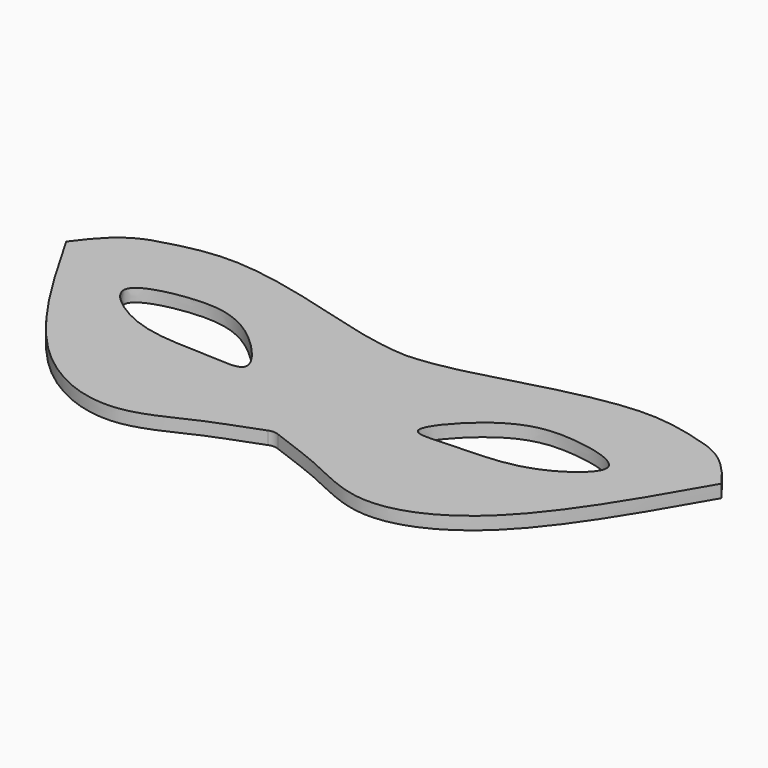
from build123d import *

# Parameters (mm, degrees)
F1_DEPTH = 2.54


with BuildPart() as f1:
    # F0 (on Top) → F1 (new body)
    with BuildSketch(Plane.XY):
        with BuildLine():
            add(Edge.make_bspline(
                [(-64.9001970887, 13.9585789293), (-59.8424235445, 21.0693185661), (-53.7346048637, 23.0257404726), (-40.3145630415, 26.4282743713), (-18.8814266067, 21.0659037421), (-6.7937120551, 17.3061378378), (0, 16.9809884228)],
                knots=[0, 0, 0, 0, 0.236178933, 0.4480704868, 0.7301373435, 1, 1, 1, 1], degree=3))
            add(Edge.make_bspline(
                [(-64.9001970887, 13.9585789293), (-60.7131418232, 6.874283925), (-47.3204689226, -18.4135182685), (-25.1756609398, -27.5932197086), (-12.0182650538, -19.6967941746), (-3.849485648, -17.1576407451), (-0.9746632453, -15.96304804)],
                knots=[0, 0, 0, 0, 0.3337918688, 0.5942910183, 0.8077332916, 0.9798868813, 0.9798868813, 0.9798868813, 0.9798868813], degree=3))
            add(Edge.make_bspline(
                [(-0.9746632453, -15.96304804), (-0.6387908173, -15.8234808959), (-0.3134590553, -15.6830816698), (0, -15.541062241)],
                knots=[0.9798868813, 0.9798868813, 0.9798868813, 0.9798868813, 1, 1, 1, 1], degree=3))
            add(Edge.make_bspline(
                [(0.9746632453, -15.96304804), (0.6387908173, -15.8234808959), (0.3134590553, -15.6830816698), (0, -15.541062241)],
                knots=[0.9798868813, 0.9798868813, 0.9798868813, 0.9798868813, 1, 1, 1, 1], degree=3))
            add(Edge.make_bspline(
                [(64.9001970887, 13.9585789293), (60.7131418232, 6.874283925), (47.3204689226, -18.4135182685), (25.1756609398, -27.5932197086), (12.0182650538, -19.6967941746), (3.849485648, -17.1576407451), (0.9746632453, -15.96304804)],
                knots=[0, 0, 0, 0, 0.3337918688, 0.5942910183, 0.8077332916, 0.9798868813, 0.9798868813, 0.9798868813, 0.9798868813], degree=3))
            add(Edge.make_bspline(
                [(64.9001970887, 13.9585789293), (59.8424235445, 21.0693185661), (53.7346048637, 23.0257404726), (40.3145630415, 26.4282743713), (18.8814266067, 21.0659037421), (6.7937120551, 17.3061378378), (0, 16.9809884228)],
                knots=[0, 0, 0, 0, 0.236178933, 0.4480704868, 0.7301373435, 1, 1, 1, 1], degree=3))
        make_face()
        with BuildLine():
            add(Edge.make_bspline(
                [(-47.7647706866, 7.2845630348), (-47.2238090705, 9.4418665585), (-36.443945915, 12.1785918421), (-25.3808361667, 10.3769526965), (-13.4196607123, -3.1638753962), (-24.0941982433, -1.8972065882), (-32.4275500412, -2.0995535899), (-41.7821849404, -0.0363742902), (-48.2414855386, 5.383469502), (-47.7647706866, 7.2845630348)],
                knots=[0, 0, 0, 0, 0.1486904868, 0.3142704588, 0.4735401823, 0.5857095329, 0.7237633974, 0.8689685898, 1, 1, 1, 1], degree=3))
        make_face(mode=Mode.SUBTRACT)
        with BuildLine():
            add(Edge.make_bspline(
                [(47.7647706866, 7.2845630348), (47.2238090705, 9.4418665585), (36.443945915, 12.1785918421), (25.3808361667, 10.3769526965), (13.4196607123, -3.1638753962), (24.0941982433, -1.8972065882), (32.4275500412, -2.0995535899), (41.7821849404, -0.0363742902), (48.2414855386, 5.383469502), (47.7647706866, 7.2845630348)],
                knots=[0, 0, 0, 0, 0.1486904868, 0.3142704588, 0.4735401823, 0.5857095329, 0.7237633974, 0.8689685898, 1, 1, 1, 1], degree=3))
        make_face(mode=Mode.SUBTRACT)
        with BuildLine():
            add(Edge.make_bspline(
                [(-0.9746632453, -15.96304804), (-0.6387908173, -15.8234808959), (-0.3134590553, -15.6830816698), (0, -15.541062241)],
                knots=[0.9798868813, 0.9798868813, 0.9798868813, 0.9798868813, 1, 1, 1, 1], degree=3))
            ThreePointArc((-0.9746632453, -15.96304804), (0, -15.7686037435), (0.9746632453, -15.96304804))
            add(Edge.make_bspline(
                [(0.9746632453, -15.96304804), (0.6387908173, -15.8234808959), (0.3134590553, -15.6830816698), (0, -15.541062241)],
                knots=[0.9798868813, 0.9798868813, 0.9798868813, 0.9798868813, 1, 1, 1, 1], degree=3))
        make_face()
    extrude(amount=F1_DEPTH)


solid = f1.part
